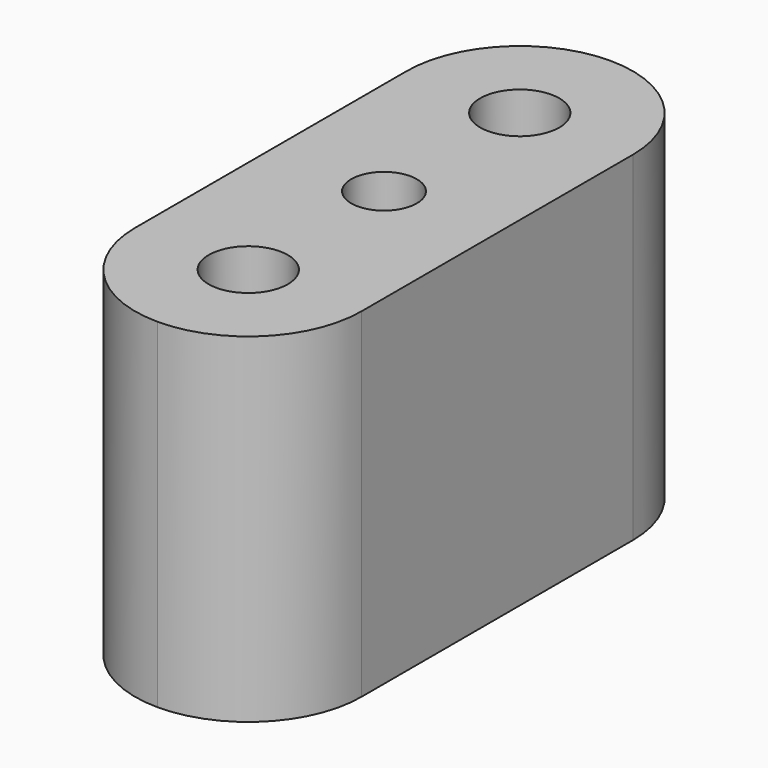
from build123d import *

# Parameters (mm, degrees)
F0_W     = 10
F0_H     = 25
F0_R     = 1.75
F0_R_2   = 1.45
F1_DEPTH = 15
F2_R     = 4.99999


# Not quite as in the source:
# - a fillet or chamfer is up to 0.001 mm smaller than in the source, because OpenCascade refuses the exact size


with BuildPart() as f1:
    # F0 (on Top) → F1 (new body)
    with BuildSketch(Plane.XY):
        Rectangle(F0_W, F0_H)
        with Locations((0, -7.5)):
            Circle(F0_R, mode=Mode.SUBTRACT)
        Circle(F0_R_2, mode=Mode.SUBTRACT)
        with Locations((0, 7.5)):
            Circle(F0_R, mode=Mode.SUBTRACT)
    extrude(amount=F1_DEPTH)

    # F2 (radius 5 in the source; OpenCascade refuses exactly that, so slightly less here)
    f2_edges = [f1.edges().sort_by_distance(p)[0] for p in [
        (-5, -12.5, 7.5),
        (5, -12.5, 7.5),
        (-5, 12.5, 7.5),
        (5, 12.5, 7.5),
    ]]
    fillet(f2_edges, radius=F2_R)


solid = f1.part
